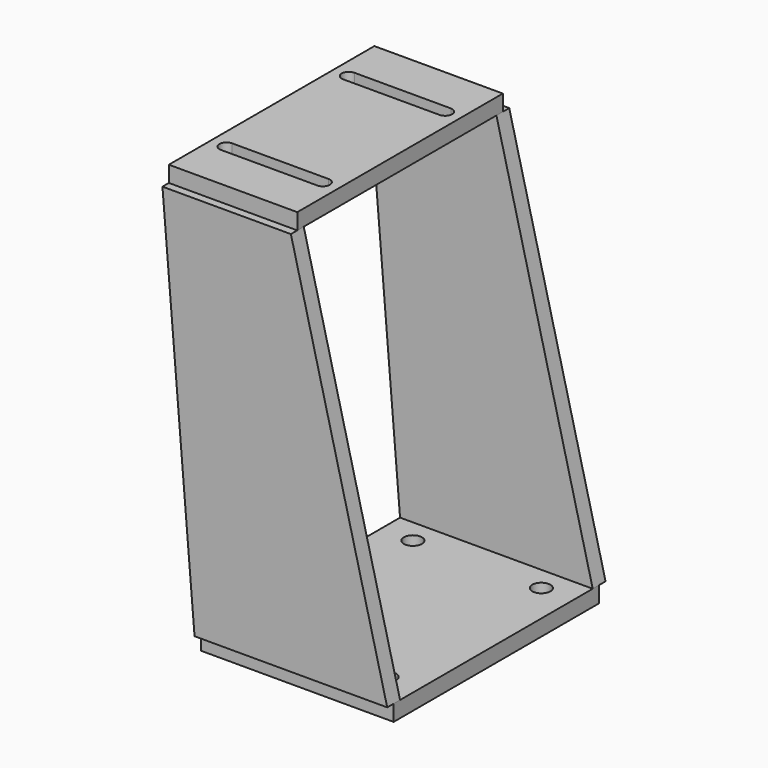
from build123d import *

# Parameters (mm, degrees)
F1_W     = 101.6
F1_H     = 203.2
F2_DEPTH = 12.7
F3_W     = 152.4
F3_H     = 203.2
F4_DEPTH = 12.7
F6_D     = 14.2875
F6_DEPTH = 50.8
F6_TIP   = 4.2923980472
F8_DEPTH = 6.35


# Not quite as in the source:
# - a length typed as a fraction of an inch, garbled in the dataset ("3 / 203.2 mm" for 3/8 in), is restored


with BuildPart() as f2:
    # F1 (on offset) → F2 (new body)
    with BuildSketch(Plane.XY.offset(330.2)):
        Rectangle(F1_W, F1_H)
        with BuildLine():
            ThreePointArc((-38.1, -66.04), (-43.688, -60.452), (-38.1, -54.864))
            Line((-38.1, -54.864), (38.1, -54.864))
            ThreePointArc((38.1, -54.864), (43.688, -60.452), (38.1, -66.04))
            Line((38.1, -66.04), (-38.1, -66.04))
        make_face(mode=Mode.SUBTRACT)
        with BuildLine():
            Line((38.1, 54.864), (-38.1, 54.864))
            ThreePointArc((-38.1, 54.864), (-43.688, 60.452), (-38.1, 66.04))
            Line((-38.1, 66.04), (38.1, 66.04))
            ThreePointArc((38.1, 66.04), (43.688, 60.452), (38.1, 54.864))
        make_face(mode=Mode.SUBTRACT)
    extrude(amount=-F2_DEPTH)



with BuildPart() as f4:
    # F3 (on Top) → F4 (new body)
    with BuildSketch(Plane.XY):
        with Locations((50.8, 0)):
            Rectangle(F3_W, F3_H)
    extrude(amount=F4_DEPTH)

    # F6
    with Locations(Plane.XY.offset(12.7)):
        with Locations((0, 76.2), (101.6, 76.2), (0, -76.2), (101.6, -76.2)):
            Hole(F6_D / 2, depth=F6_DEPTH)
            with Locations((0, 0, -(F6_DEPTH + F6_TIP / 2))):  # 118° drill point
                Cone(0, F6_D / 2, F6_TIP, mode=Mode.SUBTRACT)


with BuildPart() as f2_1:
    add(f2.part)

    add(f4.part)  # F8 merges F4
    # F7 (on face) → F8 (join, symmetric)
    with BuildSketch(Plane.XZ.offset(101.6)):
        Polygon((50.8, 317.5), (-50.8, 317.5), (-25.4, 12.7), (127, 12.7), align=None)
    extrude(amount=F8_DEPTH, both=True)

    # F9: F2 across plane


with BuildPart() as f2_2:
    add(f2_1.part)
    add(f2_1.part.mirror(Plane.XZ))


solid = f2_2.part
